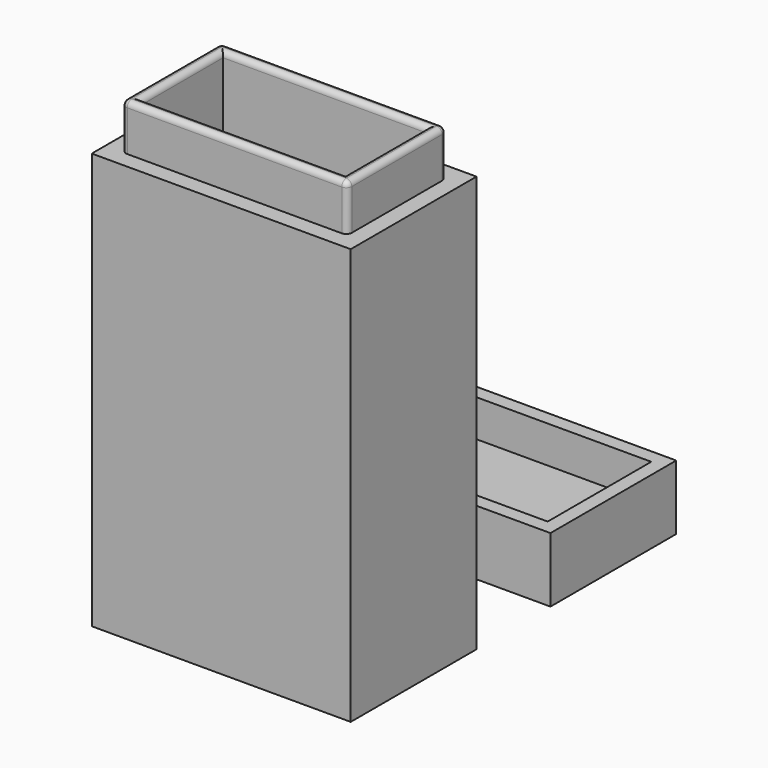
from build123d import *

# Parameters (mm, degrees)
F0_W     = 22
F0_H     = 11
F1_DEPTH = 3
F0_W_2   = 25
F0_H_2   = 14
F0_W_3   = 24.4
F0_H_3   = 13.4
F2_DEPTH = 50
F0_W_4   = 28
F0_H_4   = 17
F3_DEPTH = 45
F4_DEPTH = 7
F5_R     = 0.59999


# Not quite as in the source:
# - a fillet or chamfer is up to 0.001 mm smaller than in the source, because OpenCascade refuses the exact size


with BuildPart() as f1:
    # F0 (on Top) → F1 (new body)
    with BuildSketch(Plane.XY):
        with Locations((14, 8.5)):
            Rectangle(F0_W, F0_H)
    extrude(amount=F1_DEPTH)

    # F0 (on Top) → F2 (join)
    with BuildSketch(Plane.XY):
        with Locations((14, 8.5)):
            Rectangle(F0_W_3, F0_H_3)
        with Locations((14, 8.5)):
            Rectangle(F0_W, F0_H, mode=Mode.SUBTRACT)
    extrude(amount=F2_DEPTH)

    # F0 (on Top) → F3 (join)
    with BuildSketch(Plane.XY):
        with Locations((14, 8.5)):
            Rectangle(F0_W_4, F0_H_4)
        with Locations((14, 8.5)):
            Rectangle(F0_W_3, F0_H_3, mode=Mode.SUBTRACT)
    extrude(amount=F3_DEPTH)

    # F5 (radius 0.6 in the source; OpenCascade refuses exactly that, so slightly less here)
    f5_edges = [f1.edges().sort_by_distance(p)[0] for p in [
        (1.8, 8.5, 50),
        (14, 1.8, 50),
        (26.2, 8.5, 50),
        (14, 15.2, 50),
        (14, 3, 50),
        (3, 8.5, 50),
        (14, 14, 50),
        (25, 8.5, 50),
        (26.2, 1.8, 47.5),
        (26.2, 15.2, 47.5),
        (1.8, 15.2, 47.5),
        (1.8, 1.8, 47.5),
    ]]
    fillet(f5_edges, radius=F5_R)


with BuildPart() as f1b:
    # F0 (on Top) → F1, piece 2 (new body)
    with BuildSketch(Plane.XY):
        with Locations((14, 35.5)):
            Rectangle(F0_W_2, F0_H_2)
    extrude(amount=F1_DEPTH)

    # F0 (on Top) → F4 (join)
    with BuildSketch(Plane.XY):
        with Locations((14, 35.5)):
            Rectangle(F0_W_4, F0_H_4)
        with Locations((14, 35.5)):
            Rectangle(F0_W_2, F0_H_2, mode=Mode.SUBTRACT)
    extrude(amount=F4_DEPTH)


solid = Compound([f1.part, f1b.part])
